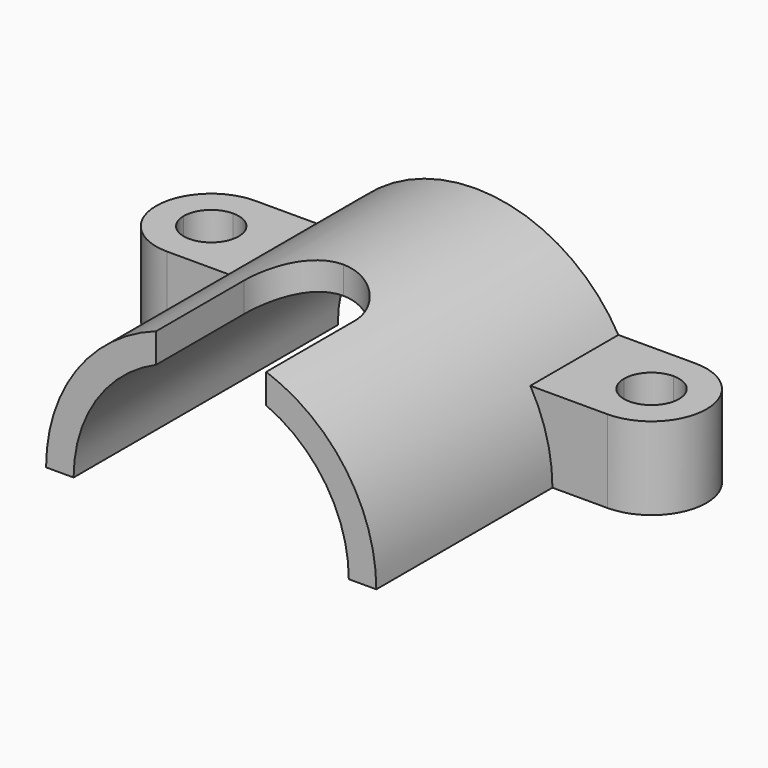
from build123d import *

# Parameters (mm, degrees)
F1_DEPTH  = 60
F3_DEPTH  = 15
F5_DEPTH  = 15.001
F7_DEPTH  = 15.001
F9_DEPTH  = 60.001
F11_REACH = 66.0565127546
F12_R     = 9.999


# Not quite as in the source:
# - a fillet or chamfer is up to 0.001 mm smaller than in the source, because OpenCascade refuses the exact size


with BuildPart() as f1:
    # F0 (on Front) → F1 (new body)
    with BuildSketch(Plane.XZ):
        with BuildLine():
            Line((-30, 0), (30, 0))
            ThreePointArc((30, 0), (0, 30), (-30, 0))
        make_face()
    extrude(amount=F1_DEPTH)

    # F2 (on face) → F3 (join)
    with BuildSketch(Plane(origin=(0, 0, 0), x_dir=(1, 0, 0), z_dir=(0, 0, -1))):
        with BuildLine():
            ThreePointArc((-40, 20), (-50, 10), (-40, 0))
            Line((-40, 0), (40, 0))
            ThreePointArc((40, 0), (50, 10), (40, 20))
            Line((40, 20), (-40, 20))
        make_face()
    extrude(amount=-F3_DEPTH)

    # F4 (on face) → F5 (cut, through all)
    with BuildSketch(Plane.XY.offset(15)):
        with BuildLine():
            Line((-45, -10), (-40, -10))
            Line((-40, -10), (-40, -5))
            ThreePointArc((-40, -5), (-43.5355339059, -6.4644660941), (-45, -10))
        make_face()
        with BuildLine():
            Line((-40, -5), (-40, -10))
            Line((-40, -10), (-35, -10))
            ThreePointArc((-35, -10), (-36.4644660941, -6.4644660941), (-40, -5))
        make_face()
        with BuildLine():
            Line((-40, -10), (-40, -15))
            ThreePointArc((-40, -15), (-36.4644660941, -13.5355339059), (-35, -10))
            Line((-35, -10), (-40, -10))
        make_face()
        with BuildLine():
            ThreePointArc((-45, -10), (-43.5355339059, -13.5355339059), (-40, -15))
            Line((-40, -15), (-40, -10))
            Line((-40, -10), (-45, -10))
        make_face()
    extrude(amount=-F5_DEPTH, mode=Mode.SUBTRACT)

    # F6 (on face) → F7 (cut, through all)
    with BuildSketch(Plane.XY.offset(15)):
        with BuildLine():
            ThreePointArc((40, -5), (36.4644660941, -6.4644660941), (35, -10))
            Line((35, -10), (40, -10))
            Line((40, -10), (40, -5))
        make_face()
        with BuildLine():
            Line((40, -5), (40, -10))
            Line((40, -10), (45, -10))
            ThreePointArc((45, -10), (43.5355339059, -6.4644660941), (40, -5))
        make_face()
        with BuildLine():
            Line((45, -10), (40, -10))
            Line((40, -10), (40, -15))
            ThreePointArc((40, -15), (43.5355339059, -13.5355339059), (45, -10))
        make_face()
        with BuildLine():
            Line((40, -10), (35, -10))
            ThreePointArc((35, -10), (36.4644660941, -13.5355339059), (40, -15))
            Line((40, -15), (40, -10))
        make_face()
    extrude(amount=-F7_DEPTH, mode=Mode.SUBTRACT)

    # F8 (on face) → F9 (cut, through all)
    with BuildSketch(Plane.XZ.offset(60)):
        with BuildLine():
            Line((-25, 0), (25, 0))
            ThreePointArc((25, 0), (0, 25), (-25, 0))
        make_face()
    extrude(amount=-F9_DEPTH, mode=Mode.SUBTRACT)

    f11_end = f1.faces().sort_by_distance((0, -30, 30))[0]
    # F10 (on Top) → F11 (cut, up to a face of the model that its end follows)
    with BuildSketch(Plane.XY):
        Polygon((-10, -60), (0, -60), (10, -60), (10, -30), (-10, -30), align=None)
    f11_long = extrude(amount=F11_REACH, mode=Mode.PRIVATE)
    add(split(f11_long, bisect_by=f11_end, keep=Keep.BOTTOM, mode=Mode.PRIVATE), mode=Mode.SUBTRACT)

    # F12 (radius 10 in the source; OpenCascade refuses exactly that, so slightly less here)
    f12_edges = [f1.edges().sort_by_distance(p)[0] for p in [
        (-10, -30, 25.598575),
        (10, -30, 25.598575),
    ]]
    fillet(f12_edges, radius=F12_R)


solid = f1.part
